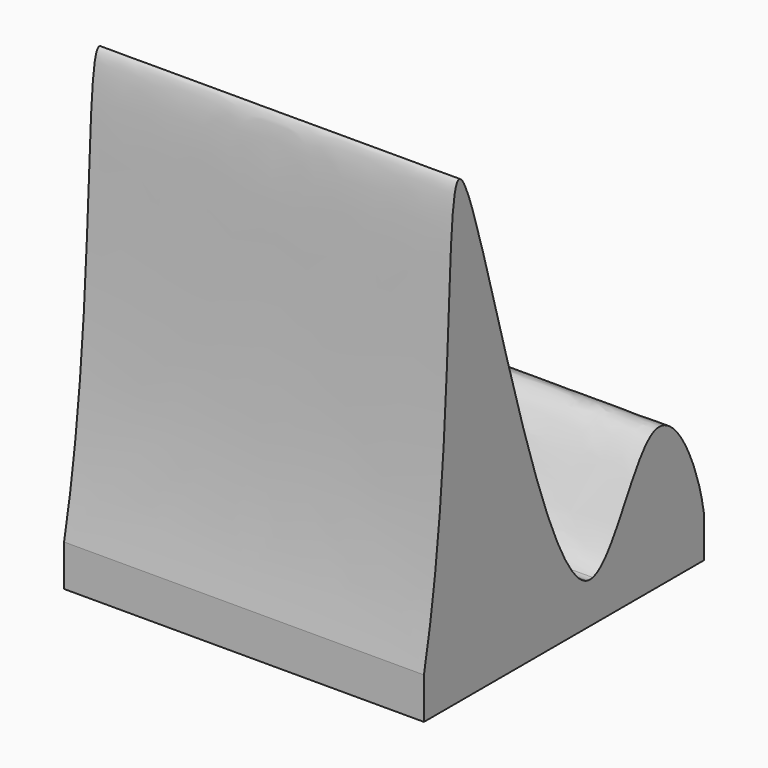
from build123d import *

# Parameters (mm, degrees)
F1_DEPTH = 65


with BuildPart() as f1:
    # F0 (on Right) → F1 (new body)
    with BuildSketch(Plane.YZ):
        with BuildLine():
            add(Edge.make_bspline(
                [(0, 0), (7.535805658, 35.7916641323), (0.7980118824, 130.0002884959), (26.7379139246, 2.4687719644), (36.8616245687, 0)],
                knots=[0, 0, 0, 0, 0.3214329284, 0.6524566012, 0.6524566012, 0.6524566012, 0.6524566012], degree=3))
            Line((0, 0), (36.8616245687, 0))
        make_face()
        with BuildLine():
            Line((36.8616245687, 0), (0, 0))
            Line((0, 0), (0, -7.4806414777))
            Line((0, -7.4806414777), (63.2124841213, -7.4806414777))
            Line((63.2124841213, -7.4806414777), (63.2124841213, 0))
            Line((63.2124841213, 0), (38.1099706596, 0))
            add(Edge.make_bspline(
                [(36.8616245687, 0), (37.2827904695, -0.1027056783), (37.6987003599, -0.097701161), (38.1099706596, 0)],
                knots=[0.6524566012, 0.6524566012, 0.6524566012, 0.6524566012, 0.6662278249, 0.6662278249, 0.6662278249, 0.6662278249], degree=3))
        make_face()
        with BuildLine():
            add(Edge.make_bspline(
                [(38.1099706596, 0), (43.0200186963, 1.1664284879), (51.645443653, 30.3569507717), (61.8684866833, 8.7077435887), (63.2124841213, 0)],
                knots=[0.6662278249, 0.6662278249, 0.6662278249, 0.6662278249, 0.8306388452, 1, 1, 1, 1], degree=3))
            Line((38.1099706596, 0), (63.2124841213, 0))
        make_face()
    extrude(amount=F1_DEPTH)


solid = f1.part
